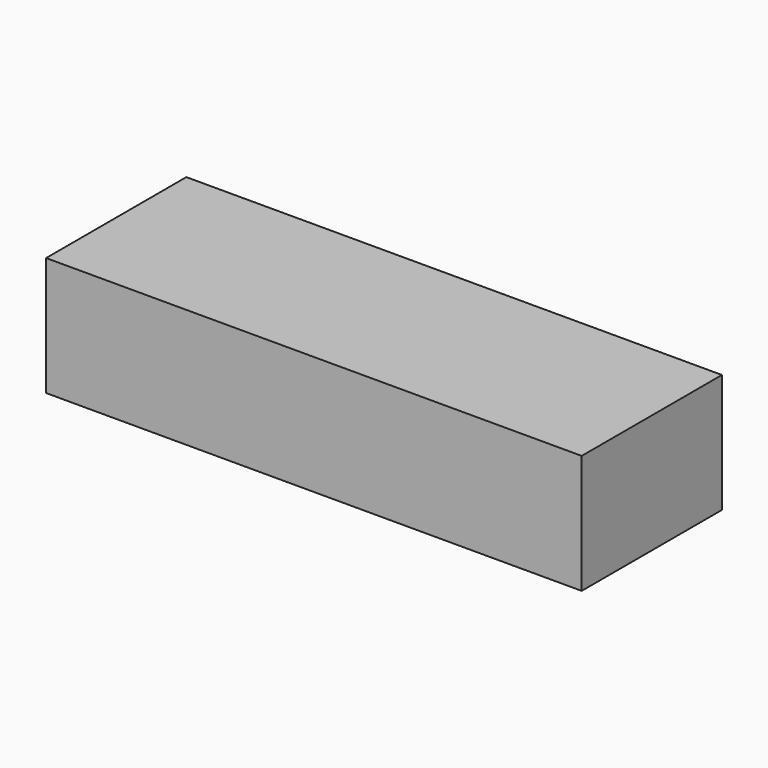
from build123d import *

# Parameters (mm, degrees)
F0_W     = 1397
F0_H     = 457.2
F1_DEPTH = 310


# Not quite as in the source:
# - a feature names something its author has since deleted; it is built from what else it names


with BuildPart() as f1:
    # F0 (on Top) → F1 (new body)
    with BuildSketch(Plane.XY):
        Rectangle(F0_W, F0_H)
    extrude(amount=F1_DEPTH)


solid = f1.part
